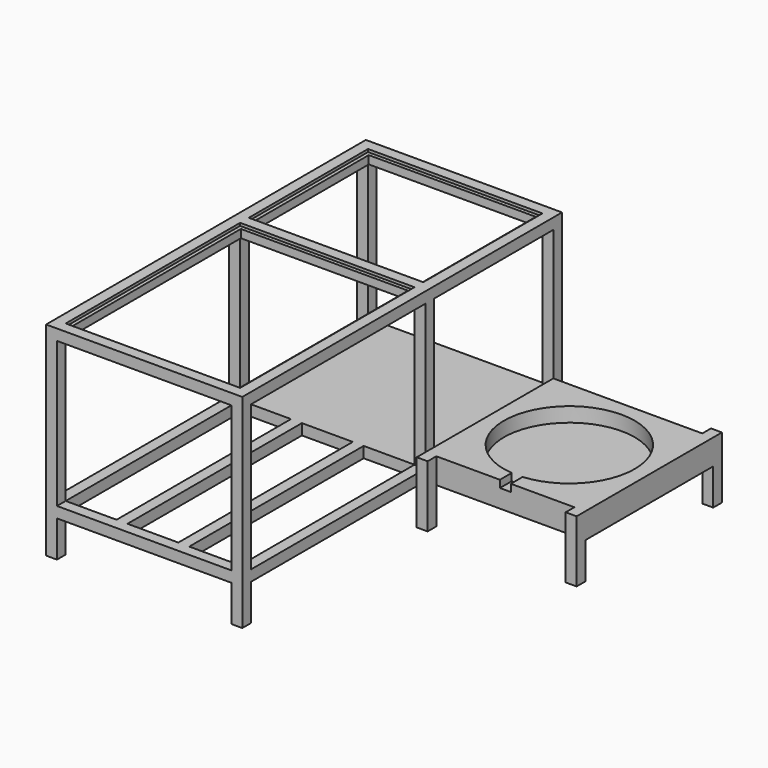
from build123d import *

# Parameters (mm, degrees)
F0_W           = 685.8
F0_H           = 1397
F1_DEPTH       = 711.2
F2_W           = 609.6
F2_H           = 508
F2_H_2         = 88.9
F3_DEPTH       = 800.1
F4_W           = 609.6
F4_H           = 88.9
F5_DEPTH       = 596.901
F6_W           = 609.6
F6_H           = 762
F7_DEPTH       = 9.525
F8_W           = 584.2
F8_H           = 736.6
F9_DEPTH       = 50.8
F10_W          = 609.6
F10_H          = 38.1
F11_DEPTH      = 1397.001
F12_W          = 762
F12_H          = 508
F12_W_2        = 1320.8
F12_H_2        = 127
F13_DEPTH      = 685.801
F14_W          = 609.6
F14_H          = 508
F15_DEPTH      = 584.2
F16_W          = 609.6
F16_H          = 520.7
F17_DEPTH      = 9.525
F18_W          = 584.2
F18_H          = 495.3
F19_DEPTH      = 28.575
F21_DEPTH      = 685.801
F22_W          = 558.8
F22_H          = 38.1
F23_DEPTH      = 558.8
F24_W          = 558.7746
F24_H          = 558.8
F24_R          = 228.6
F25_DEPTH      = 50.8
F26_W          = 38.1
F26_H          = 25.4
F27_DEPTH      = 52.5951328439
F28_W          = 38.1
F28_H          = 38.1
F29_DEPTH      = 127
F29_DEPTH_BACK = 88.9
F30_W          = 609.6
F30_H          = 508
F31_DEPTH      = 12.7
F32_W          = 609.6
F32_H          = 762
F33_DEPTH      = 165.101
F34_W          = 38.1
F34_H          = 38.1
F35_DEPTH      = 762


# Not quite as in the source:
# - a length typed as a fraction of an inch, garbled in the dataset ("3 / 203.2 mm" for 3/8 in), is restored


with BuildPart() as f1:
    # F0 (on Top) → F1 (new body)
    with BuildSketch(Plane.XY):
        Rectangle(F0_W, F0_H)
    extrude(amount=F1_DEPTH)

    # F2 (on face) → F3 (cut)
    with BuildSketch(Plane.XZ.offset(698.5)):
        with Locations((0, 419.1)):
            Rectangle(F2_W, F2_H)
        with Locations((0, 82.55)):
            Rectangle(F2_W, F2_H_2)
    extrude(amount=-F3_DEPTH, mode=Mode.SUBTRACT)

    # F4 (on face) → F5 (cut, through all)
    with BuildSketch(Plane.XZ.offset(-101.6)):
        with Locations((0, 82.55)):
            Rectangle(F4_W, F4_H)
    extrude(amount=-F5_DEPTH, mode=Mode.SUBTRACT)

    # F6 (on face) → F7 (cut)
    with BuildSketch(Plane.XY.offset(711.2)):
        with Locations((0, -279.4)):
            Rectangle(F6_W, F6_H)
    extrude(amount=-F7_DEPTH, mode=Mode.SUBTRACT)

    # F8 (on face) → F9 (cut)
    with BuildSketch(Plane.XY.offset(701.675)):
        with Locations((0, -279.4)):
            Rectangle(F8_W, F8_H)
    extrude(amount=-F9_DEPTH, mode=Mode.SUBTRACT)

    # F10 (on face) → F11 (cut, through all)
    with BuildSketch(Plane.XZ.offset(698.5)):
        with Locations((0, 19.05)):
            Rectangle(F10_W, F10_H)
    extrude(amount=-F11_DEPTH, mode=Mode.SUBTRACT)

    # F12 (on face) → F13 (cut, through all)
    with BuildSketch(Plane(origin=(-342.9, 0, 0), x_dir=(0, -1, 0), z_dir=(-1, 0, 0))):
        with Locations((279.4, 419.1)):
            Rectangle(F12_W, F12_H)
        with Locations((0, 63.5)):
            Rectangle(F12_W_2, F12_H_2)
    extrude(amount=-F13_DEPTH, mode=Mode.SUBTRACT)

    # F14 (on face) → F15 (cut)
    with BuildSketch(Plane(origin=(0, 698.5, 0), x_dir=(-1, 0, 0), z_dir=(0, 1, 0))):
        with Locations((0, 419.1)):
            Rectangle(F14_W, F14_H)
    extrude(amount=-F15_DEPTH, mode=Mode.SUBTRACT)

    # F16 (on face) → F17 (cut)
    with BuildSketch(Plane.XY.offset(711.2)):
        with Locations((0, 400.05)):
            Rectangle(F16_W, F16_H)
    extrude(amount=-F17_DEPTH, mode=Mode.SUBTRACT)

    # F18 (on face) → F19 (cut, through all)
    with BuildSketch(Plane.XY.offset(701.675)):
        with Locations((0, 400.05)):
            Rectangle(F18_W, F18_H)
    extrude(amount=-F19_DEPTH, mode=Mode.SUBTRACT)

    # F20 (on face) → F21 (cut, through all)
    with BuildSketch(Plane.YZ.offset(342.9)):
        Polygon((660.4, 673.1), (647.7, 673.1), (152.4, 673.1), (139.7, 673.1), (139.7, 165.1), (660.4, 165.1), align=None)
    extrude(amount=-F21_DEPTH, mode=Mode.SUBTRACT)

    # F22 (on face) → F23 (join)
    with BuildSketch(Plane.YZ.offset(342.9)):
        with Locations((381, 146.05)):
            Rectangle(F22_W, F22_H)
    extrude(amount=F23_DEPTH)

    # F24 (on face) → F25 (join)
    with BuildSketch(Plane.XY.offset(165.1)):
        with Locations((622.3127, 381)):
            Rectangle(F24_W, F24_H)
        with Locations((622.3, 381)):
            Circle(F24_R, mode=Mode.SUBTRACT)
    extrude(amount=F25_DEPTH)

    # F26 (on face) → F27 (cut, up to face)
    with BuildSketch(Plane.XZ.offset(-101.6)):
        with Locations((622.3, 203.2)):
            Rectangle(F26_W, F26_H)
    extrude(amount=-F27_DEPTH, mode=Mode.SUBTRACT)

    # F28 (on face) → F29 (join, two sides)
    with BuildSketch(Plane(origin=(0, 0, 127), x_dir=(1, 0, 0), z_dir=(0, 0, -1))) as f29_sk:
        with Locations((882.65, -82.55)):
            Rectangle(F28_W, F28_H)
        with Locations((882.65, -679.45)):
            Rectangle(F28_W, F28_H)
        with Locations((361.9619884968, -82.55)):
            Rectangle(F28_W, F28_H)
    extrude(amount=F29_DEPTH)
    extrude(f29_sk.sketch, amount=-F29_DEPTH_BACK)

    # F30 (on face) → F31 (cut, through all)
    with BuildSketch(Plane(origin=(0, 114.3, 0), x_dir=(-1, 0, 0), z_dir=(0, 1, 0))):
        with Locations((0, 419.1)):
            Rectangle(F30_W, F30_H)
    extrude(amount=-F31_DEPTH, mode=Mode.SUBTRACT)

    # F32 (on face) → F33 (cut, through all)
    with BuildSketch(Plane.XY.offset(165.1)):
        with Locations((0, -279.4)):
            Rectangle(F32_W, F32_H)
    extrude(amount=-F33_DEPTH, mode=Mode.SUBTRACT)

    # F34 (on face) → F35 (join, through all)
    with BuildSketch(Plane.XZ.offset(-101.6)):
        with Locations((107.95, 146.05)):
            Rectangle(F34_W, F34_H)
        with Locations((-107.95, 146.05)):
            Rectangle(F34_W, F34_H)
    extrude(amount=F35_DEPTH)


solid = f1.part
